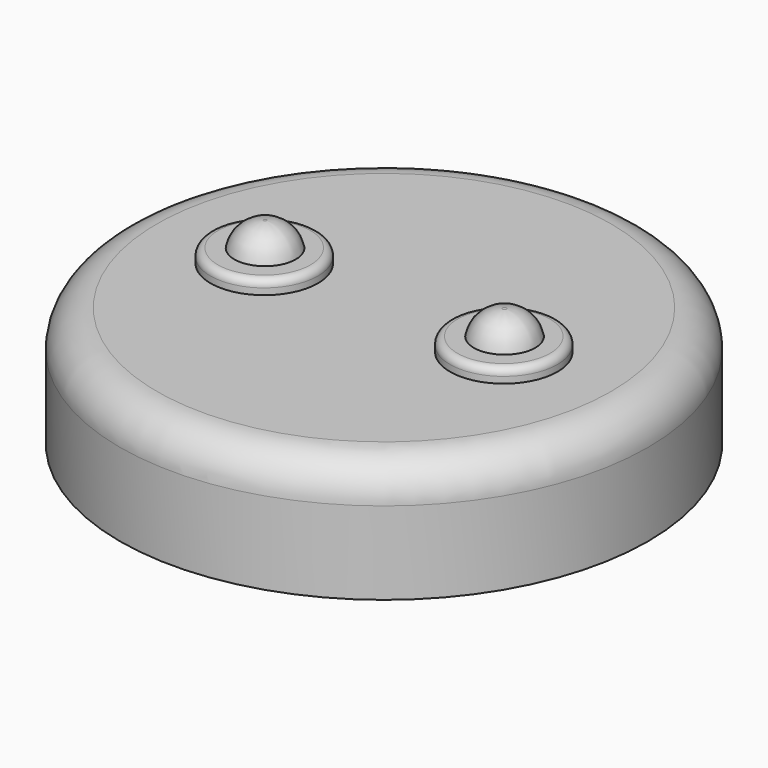
from build123d import *

# Parameters (mm, degrees)
F0_R     = 4.3688
F1_DEPTH = 1.9812
F2_R     = 0.889
F3_DEPTH = 2.2098
F4_R     = 0.508
F5_DEPTH = 2.6162
F8_R     = 0.122642049
F9_R     = 0.6132102448


# Not quite as in the source:
# - a fillet or chamfer that OpenCascade refuses, or shapes differently, is made with other operations: its cross-section is extruded or revolved along the edge and cut away or added


with BuildPart() as f1:
    # F0 (on Top) → F1 (new body)
    with BuildSketch(Plane.XY):
        Circle(F0_R)
    extrude(amount=F1_DEPTH)

    # F2 (on Top) → F3 (join)
    with BuildSketch(Plane.XY):
        with Locations((-1.9812, 0)):
            Circle(F2_R)
        with Locations((1.9812, 0)):
            Circle(F2_R)
    extrude(amount=F3_DEPTH)

    # F4 (on Top) → F5 (join)
    with BuildSketch(Plane.XY):
        with Locations((-1.9675190561, 0)):
            Circle(F4_R)
        with Locations((1.9938375335, 0)):
            Circle(F4_R)
    extrude(amount=F5_DEPTH)

    # F6: fillet of radius 0.4905681959 on 1 edges, made by hand

    # F6_s1 → F6_t2 (revolve, cut)
    with BuildSketch(Plane.XZ):
        with BuildLine():
            ThreePointArc((-1.4595190561, 2.2098), (-1.6270859561, 2.5010964461), (-1.9428128276, 2.6162))
            Line((-1.9428128276, 2.6162), (-1.4595190561, 2.6162))
            Line((-1.4595190561, 2.6162), (-1.4595190561, 2.2098))
        make_face()
    revolve(axis=Axis((-1.9675190561, 0, 2.6162), (0, 0, 1)), mode=Mode.SUBTRACT)

    # F7: fillet of radius 0.4826 on 1 edges, made by hand

    # F7_s1 → F7_t2 (revolve, cut)
    with BuildSketch(Plane.XZ):
        with BuildLine():
            ThreePointArc((2.5018375335, 2.2098), (2.3384435237, 2.5008035403), (2.0252912923, 2.6162))
            Line((2.0252912923, 2.6162), (2.5018375335, 2.6162))
            Line((2.5018375335, 2.6162), (2.5018375335, 2.2098))
        make_face()
    revolve(axis=Axis((1.9938375335, 0, 2.6162), (0, 0, 1)), mode=Mode.SUBTRACT)

    # F8
    f8_edges = [f1.edges().sort_by_distance(p)[0] for p in [
        (-2.8702, 0, 2.2098),
        (1.0922, 0, 2.2098),
    ]]
    fillet(f8_edges, radius=F8_R)

    # F9
    f9_edges = [f1.edges().sort_by_distance(p)[0] for p in [
        (-4.3688, 0, 1.9812),
    ]]
    fillet(f9_edges, radius=F9_R)


solid = f1.part
